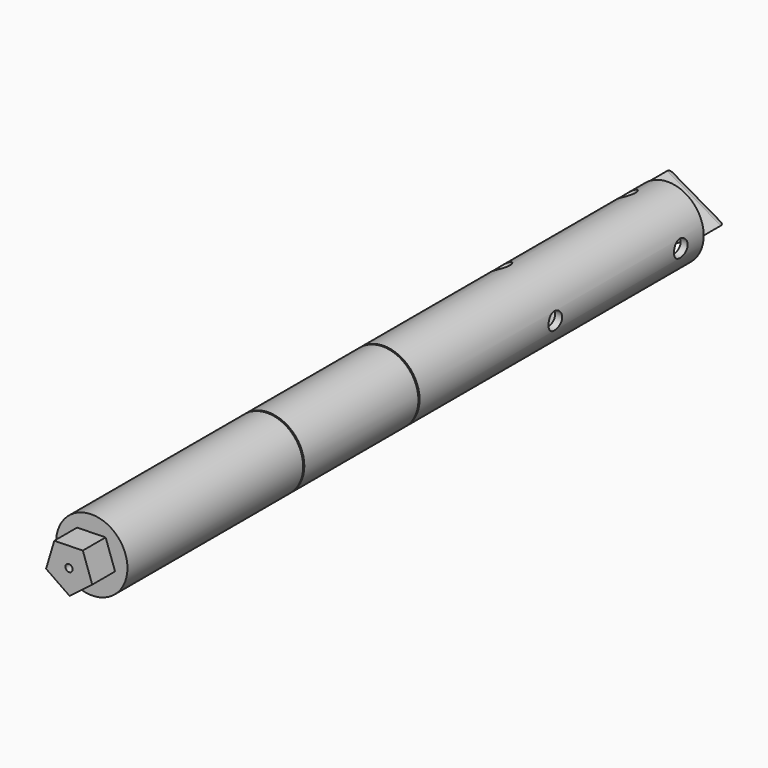
from build123d import *

# Parameters (mm, degrees)
F0_R      = 25
F0_R_2    = 20
F1_DEPTH  = 500
F2_R      = 25
F3_DEPTH  = 5
F5_DEPTH  = 20
F7_D      = 5
F10_D     = 12
F10_DEPTH = 6
F10_START = 0.7306779
F10_TIP   = 3.6051637142
F12_DEPTH = 20
F17_D     = 12
F17_DEPTH = 6
F17_START = 0.7306779
F17_TIP   = 3.6051637142
F19_D     = 12
F19_DEPTH = 6
F19_START = 0.7306779
F19_TIP   = 3.6051637142
F20_R     = 5
F22_R     = 25
F22_R_2   = 24
F23_DEPTH = 1
F25_R     = 25
F25_R_2   = 24
F26_DEPTH = 1


with BuildPart() as f1:
    # F0 (on Front) → F1 (new body)
    with BuildSketch(Plane.XZ):
        Circle(F0_R)
        Circle(F0_R_2, mode=Mode.SUBTRACT)
    extrude(amount=F1_DEPTH)

    # F2 (on face) → F3 (join)
    with BuildSketch(Plane.XZ.offset(500)):
        Circle(F2_R)
    extrude(amount=F3_DEPTH)

    # F4 (on face) → F5 (join)
    with BuildSketch(Plane.XZ.offset(505)):
        Polygon((-16.0628025015, -5.6190539991), (0.380358971, -17.013016167), (16.2978772735, -4.8955682433), (9.6922831285, 13.9873885984), (-10.3077168715, 13.540249811), align=None)
    extrude(amount=F5_DEPTH)

    # F7 (through all)
    with Locations(Plane.XZ.offset(525)):
        with Locations((0, 0)):
            Hole(F7_D / 2)

    # F10
    # its depths count from where the whole tool has entered the part; down to there all is cleared
    with Locations(Plane.YZ.offset(25).offset(-F10_START)):
        with Locations((-20, 0), (-130, 0)):
            Hole(F10_D / 2, depth=F10_DEPTH)
            with Locations((0, 0, -(F10_DEPTH + F10_TIP / 2))):  # 118° drill point
                Cone(0, F10_D / 2, F10_TIP, mode=Mode.SUBTRACT)

    # F11 (on face) → F12 (join)
    with BuildSketch(Plane(origin=(0, 0, 0), x_dir=(-1, 0, 0), z_dir=(0, 1, 0))):
        Polygon((12.5, -21.6506350946), (12.5, 21.6506350946), (-25, 0), align=None)
    extrude(amount=F12_DEPTH)

    # F17
    # its depths count from where the whole tool has entered the part; down to there all is cleared
    with Locations(Plane(origin=(-12.5, 0, -21.6506350946), x_dir=(0.8660254038, 0, -0.5), z_dir=(-0.5, 0, -0.8660254038)).offset(-F17_START)):
        with Locations((0, 20), (0, 130)):
            Hole(F17_D / 2, depth=F17_DEPTH)
            with Locations((0, 0, -(F17_DEPTH + F17_TIP / 2))):  # 118° drill point
                Cone(0, F17_D / 2, F17_TIP, mode=Mode.SUBTRACT)

    # F19
    # its depths count from where the whole tool has entered the part; down to there all is cleared
    with Locations(Plane(origin=(-12.5, 0, 21.6506350946), x_dir=(0.8660254038, 0, 0.5), z_dir=(-0.5, 0, 0.8660254038)).offset(-F19_START)):
        with Locations((0, -20), (0, -130)):
            Hole(F19_D / 2, depth=F19_DEPTH)
            with Locations((0, 0, -(F19_DEPTH + F19_TIP / 2))):  # 118° drill point
                Cone(0, F19_D / 2, F19_TIP, mode=Mode.SUBTRACT)

    # F20
    f20_edges = [f1.edges().sort_by_distance(p)[0] for p in [
        (6.25, 20, 10.825318),
        (-12.5, 20, 0),
        (6.25, 20, -10.825318),
    ]]
    fillet(f20_edges, radius=F20_R)

    # F22 (on offset) → F23 (cut)
    with BuildSketch(Plane.XZ.offset(250)):
        Circle(F22_R)
        Circle(F22_R_2, mode=Mode.SUBTRACT)
    extrude(amount=-F23_DEPTH, mode=Mode.SUBTRACT)

    # F25 (on offset) → F26 (cut)
    with BuildSketch(Plane.XZ.offset(350)):
        Circle(F25_R)
        Circle(F25_R_2, mode=Mode.SUBTRACT)
    extrude(amount=F26_DEPTH, mode=Mode.SUBTRACT)


solid = f1.part
